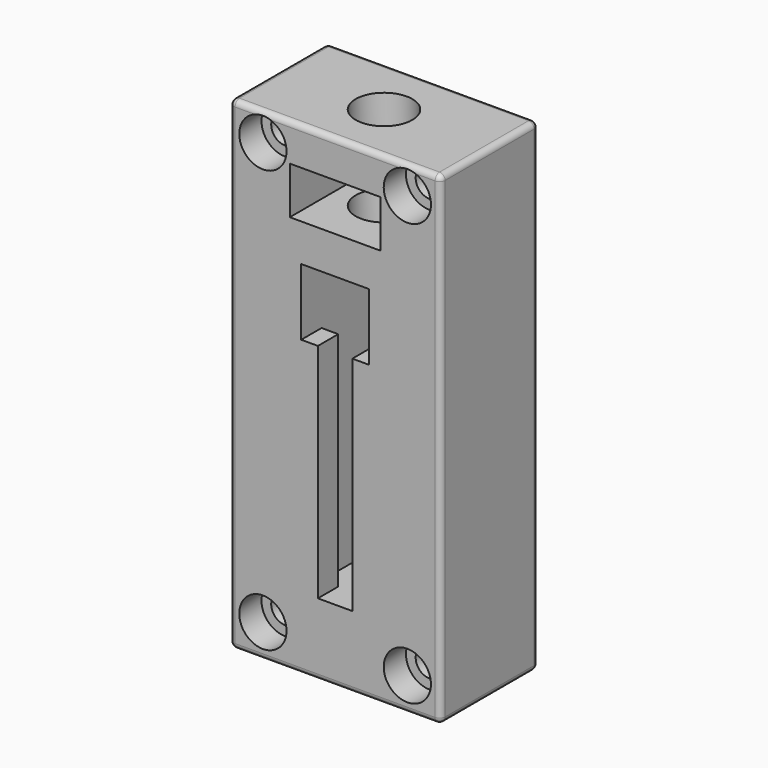
from build123d import *

# Parameters (mm, degrees)
F0_W         = 16.3
F0_H         = 8.5
F1_DEPTH     = 22
F2_R         = 5.1
F3_DEPTH     = 22
F4_W         = 3
F4_H         = 12.2
F4_W_2       = 9.2
F5_DEPTH     = 40
F6_R         = 2.5
F7_DEPTH     = 22.001
F6_R_2       = 4.25
F8_DEPTH     = 5
F9_T1_DEPTH  = 85
F9_T3_DEPTH  = 36
F9_T5_DEPTH  = 20
F9_S9_W      = 1
F9_S9_H      = 1
F9_T10_DEPTH = 1
F9_S15_W     = 1
F9_S15_H     = 1
F9_T16_DEPTH = 1
F9_S21_W     = 1
F9_S21_H     = 1
F9_T22_DEPTH = 1
F9_S27_W     = 1
F9_S27_H     = 1
F9_T28_DEPTH = 1
F9_S33_W     = 1
F9_S33_H     = 1
F9_T34_DEPTH = 1
F9_S39_W     = 1
F9_S39_H     = 1
F9_T40_DEPTH = 1
F9_S45_W     = 1
F9_S45_H     = 1
F9_T46_DEPTH = 1
F9_S51_W     = 1
F9_S51_H     = 1
F9_T52_DEPTH = 1


# Not quite as in the source:
# - a fillet or chamfer that OpenCascade refuses, or shapes differently, is made with other operations: its cross-section is extruded or revolved along the edge and cut away or added


with BuildPart() as f1:
    # F0 (on Front) → F1 (new body)
    with BuildSketch(Plane.XZ):
        Polygon((-19, 32), (-6.1, 32), (6.1, 32), (19, 32), (19, 54), (-19, 54), align=None)
        with Locations((0, 43)):
            Rectangle(F0_W, F0_H, mode=Mode.SUBTRACT)
        Polygon((-3.1, -20), (-3.1, 20), (-6.1, 20), (-6.1, 32), (-19, 32), (-19, -33), (19, -33), (19, 32), (6.1, 32), (6.1, 20), (3.1, 20), (3.1, -20), align=None)
    extrude(amount=F1_DEPTH)

    # F2 (on face) → F3 (cut, through all)
    with BuildSketch(Plane.XY.offset(54)):
        with Locations((0, -11)):
            Circle(F2_R)
    extrude(amount=-F3_DEPTH, mode=Mode.SUBTRACT)

    # F4 (on face) → F5 (cut)
    with BuildSketch(Plane.XY.offset(20)):
        with Locations((-4.6, -11.319772105)):
            Rectangle(F4_W, F4_H)
        with Locations((1.5, -11.319772105)):
            Rectangle(F4_W_2, F4_H)
    extrude(amount=-F5_DEPTH, mode=Mode.SUBTRACT)

    # F6 (on face) → F7 (cut, through all)
    with BuildSketch(Plane.XZ.offset(22)):
        with Locations((-13, 49)):
            Circle(F6_R)
        with Locations((13, 49)):
            Circle(F6_R)
        with Locations((-13, -27)):
            Circle(F6_R)
        with Locations((13, -27)):
            Circle(F6_R)
    extrude(amount=-F7_DEPTH, mode=Mode.SUBTRACT)

    # F6 (on face) → F8 (cut)
    with BuildSketch(Plane.XZ.offset(22)):
        with Locations((-13, 49)):
            Circle(F6_R_2)
        with Locations((-13, 49)):
            Circle(F6_R, mode=Mode.SUBTRACT)
        with Locations((13, 49)):
            Circle(F6_R_2)
        with Locations((13, 49)):
            Circle(F6_R, mode=Mode.SUBTRACT)
        with Locations((13, -27)):
            Circle(F6_R_2)
        with Locations((13, -27)):
            Circle(F6_R, mode=Mode.SUBTRACT)
        with Locations((-13, -27)):
            Circle(F6_R_2)
        with Locations((-13, -27)):
            Circle(F6_R, mode=Mode.SUBTRACT)
    extrude(amount=-F8_DEPTH, mode=Mode.SUBTRACT)

    # F9: fillet of radius 1 on 12 edges, made by hand

    # F9_s2 → F9_t1 (cut)
    with BuildSketch(Plane.XY.offset(-32)):
        with BuildLine():
            ThreePointArc((18, -22), (18.7071067812, -21.7071067812), (19, -21))
            Line((19, -21), (19, -22))
            Line((19, -22), (18, -22))
        make_face()
        with BuildLine():
            ThreePointArc((-18, -22), (-18.7071067812, -21.7071067812), (-19, -21))
            Line((-19, -21), (-19, -22))
            Line((-19, -22), (-18, -22))
        make_face()
        with BuildLine():
            ThreePointArc((-18, 0), (-18.7071067812, -0.2928932188), (-19, -1))
            Line((-19, -1), (-19, 0))
            Line((-19, 0), (-18, 0))
        make_face()
        with BuildLine():
            ThreePointArc((18, 0), (18.7071067812, -0.2928932188), (19, -1))
            Line((19, -1), (19, 0))
            Line((19, 0), (18, 0))
        make_face()
    extrude(amount=F9_T1_DEPTH, mode=Mode.SUBTRACT)

    # F9_s4 → F9_t3 (cut)
    with BuildSketch(Plane.YZ.offset(-18)):
        with BuildLine():
            ThreePointArc((-22, 53), (-21.7071067812, 53.7071067812), (-21, 54))
            Line((-21, 54), (-22, 54))
            Line((-22, 54), (-22, 53))
        make_face()
        with BuildLine():
            ThreePointArc((-22, -32), (-21.7071067812, -32.7071067812), (-21, -33))
            Line((-21, -33), (-22, -33))
            Line((-22, -33), (-22, -32))
        make_face()
        with BuildLine():
            ThreePointArc((0, 53), (-0.2928932188, 53.7071067812), (-1, 54))
            Line((-1, 54), (0, 54))
            Line((0, 54), (0, 53))
        make_face()
        with BuildLine():
            ThreePointArc((0, -32), (-0.2928932188, -32.7071067812), (-1, -33))
            Line((-1, -33), (0, -33))
            Line((0, -33), (0, -32))
        make_face()
    extrude(amount=F9_T3_DEPTH, mode=Mode.SUBTRACT)

    # F9_s6 → F9_t5 (cut)
    with BuildSketch(Plane.XZ.offset(1)):
        with BuildLine():
            ThreePointArc((19, -32), (18.7071067812, -32.7071067812), (18, -33))
            Line((18, -33), (19, -33))
            Line((19, -33), (19, -32))
        make_face()
        with BuildLine():
            ThreePointArc((18, 54), (18.7071067812, 53.7071067812), (19, 53))
            Line((19, 53), (19, 54))
            Line((19, 54), (18, 54))
        make_face()
        with BuildLine():
            ThreePointArc((-18, 54), (-18.7071067812, 53.7071067812), (-19, 53))
            Line((-19, 53), (-19, 54))
            Line((-19, 54), (-18, 54))
        make_face()
        with BuildLine():
            ThreePointArc((-19, -32), (-18.7071067812, -32.7071067812), (-18, -33))
            Line((-18, -33), (-19, -33))
            Line((-19, -33), (-19, -32))
        make_face()
    extrude(amount=F9_T5_DEPTH, mode=Mode.SUBTRACT)


with BuildPart() as f9_tool8:
    # F9_s9 → F9_t10 (new body)
    with BuildSketch(Plane.XZ.offset(21)):
        with Locations((18.5, -32.5)):
            Rectangle(F9_S9_W, F9_S9_H)
    extrude(amount=F9_T10_DEPTH)

    # F9_s11 → F9_t12 (revolve, cut)
    with BuildSketch(Plane(origin=(18, -21, -32), x_dir=(-0.7071067812, 0, 0.7071067812), z_dir=(0.7071067812, 0, 0.7071067812))):
        with BuildLine():
            ThreePointArc((0, -1), (1, 0), (0, 1))
            Line((0, 1), (0, -1))
        make_face()
    revolve(axis=Axis((18, -21, -32), (0, -1, 0)), mode=Mode.SUBTRACT)


with BuildPart() as f1_1:
    add(f1.part)

    # F9_t7: cut F9_tool8
    add(f9_tool8.part, mode=Mode.SUBTRACT)


with BuildPart() as f9_tool14:
    # F9_s15 → F9_t16 (new body)
    with BuildSketch(Plane.XY.offset(53)):
        with Locations((18.5, -21.5)):
            Rectangle(F9_S15_W, F9_S15_H)
    extrude(amount=F9_T16_DEPTH)

    # F9_s17 → F9_t18 (revolve, cut)
    with BuildSketch(Plane(origin=(18, -21, 53), x_dir=(-0.7071067812, 0.7071067812, 0), z_dir=(0.7071067812, 0.7071067812, 0))):
        with BuildLine():
            ThreePointArc((0, -1), (1, 0), (0, 1))
            Line((0, 1), (0, -1))
        make_face()
    revolve(axis=Axis((18, -21, 53), (0, 0, 1)), mode=Mode.SUBTRACT)


with BuildPart() as f1_2:
    add(f1_1.part)

    # F9_t13: cut F9_tool14
    add(f9_tool14.part, mode=Mode.SUBTRACT)


with BuildPart() as f9_tool20:
    # F9_s21 → F9_t22 (new body)
    with BuildSketch(Plane.XY.offset(53)):
        with Locations((-18.5, -21.5)):
            Rectangle(F9_S21_W, F9_S21_H)
    extrude(amount=F9_T22_DEPTH)

    # F9_s23 → F9_t24 (revolve, cut)
    with BuildSketch(Plane(origin=(-18, -21, 53), x_dir=(0.7071067812, 0.7071067812, 0), z_dir=(0.7071067812, -0.7071067812, 0))):
        with BuildLine():
            ThreePointArc((0, -1), (1, 0), (0, 1))
            Line((0, 1), (0, -1))
        make_face()
    revolve(axis=Axis((-18, -21, 53), (0, 0, 1)), mode=Mode.SUBTRACT)


with BuildPart() as f1_3:
    add(f1_2.part)

    # F9_t19: cut F9_tool20
    add(f9_tool20.part, mode=Mode.SUBTRACT)


with BuildPart() as f9_tool26:
    # F9_s27 → F9_t28 (new body)
    with BuildSketch(Plane.XZ.offset(21)):
        with Locations((-18.5, -32.5)):
            Rectangle(F9_S27_W, F9_S27_H)
    extrude(amount=F9_T28_DEPTH)

    # F9_s29 → F9_t30 (revolve, cut)
    with BuildSketch(Plane(origin=(-18, -21, -32), x_dir=(0.7071067812, 0, 0.7071067812), z_dir=(0.7071067812, 0, -0.7071067812))):
        with BuildLine():
            ThreePointArc((0, -1), (1, 0), (0, 1))
            Line((0, 1), (0, -1))
        make_face()
    revolve(axis=Axis((-18, -21, -32), (0, -1, 0)), mode=Mode.SUBTRACT)


with BuildPart() as f1_4:
    add(f1_3.part)

    # F9_t25: cut F9_tool26
    add(f9_tool26.part, mode=Mode.SUBTRACT)


with BuildPart() as f9_tool32:
    # F9_s33 → F9_t34 (new body)
    with BuildSketch(Plane.XZ.offset(1)):
        with Locations((18.5, -32.5)):
            Rectangle(F9_S33_W, F9_S33_H)
    extrude(amount=-F9_T34_DEPTH)

    # F9_s35 → F9_t36 (revolve, cut)
    with BuildSketch(Plane(origin=(18, -1, -32), x_dir=(-0.7071067812, 0, 0.7071067812), z_dir=(-0.7071067812, 0, -0.7071067812))):
        with BuildLine():
            ThreePointArc((0, -1), (1, 0), (0, 1))
            Line((0, 1), (0, -1))
        make_face()
    revolve(axis=Axis((18, -1, -32), (0, 1, 0)), mode=Mode.SUBTRACT)


with BuildPart() as f1_5:
    add(f1_4.part)

    # F9_t31: cut F9_tool32
    add(f9_tool32.part, mode=Mode.SUBTRACT)


with BuildPart() as f9_tool38:
    # F9_s39 → F9_t40 (new body)
    with BuildSketch(Plane.XZ.offset(1)):
        with Locations((18.5, 53.5)):
            Rectangle(F9_S39_W, F9_S39_H)
    extrude(amount=-F9_T40_DEPTH)

    # F9_s41 → F9_t42 (revolve, cut)
    with BuildSketch(Plane(origin=(18, -1, 53), x_dir=(-0.7071067812, 0, -0.7071067812), z_dir=(0.7071067812, 0, -0.7071067812))):
        with BuildLine():
            ThreePointArc((0, -1), (1, 0), (0, 1))
            Line((0, 1), (0, -1))
        make_face()
    revolve(axis=Axis((18, -1, 53), (0, 1, 0)), mode=Mode.SUBTRACT)


with BuildPart() as f1_6:
    add(f1_5.part)

    # F9_t37: cut F9_tool38
    add(f9_tool38.part, mode=Mode.SUBTRACT)


with BuildPart() as f9_tool44:
    # F9_s45 → F9_t46 (new body)
    with BuildSketch(Plane.XZ.offset(1)):
        with Locations((-18.5, 53.5)):
            Rectangle(F9_S45_W, F9_S45_H)
    extrude(amount=-F9_T46_DEPTH)

    # F9_s47 → F9_t48 (revolve, cut)
    with BuildSketch(Plane(origin=(-18, -1, 53), x_dir=(0.7071067812, 0, -0.7071067812), z_dir=(0.7071067812, 0, 0.7071067812))):
        with BuildLine():
            ThreePointArc((0, -1), (1, 0), (0, 1))
            Line((0, 1), (0, -1))
        make_face()
    revolve(axis=Axis((-18, -1, 53), (0, 1, 0)), mode=Mode.SUBTRACT)


with BuildPart() as f1_7:
    add(f1_6.part)

    # F9_t43: cut F9_tool44
    add(f9_tool44.part, mode=Mode.SUBTRACT)


with BuildPart() as f9_tool50:
    # F9_s51 → F9_t52 (new body)
    with BuildSketch(Plane.XZ.offset(1)):
        with Locations((-18.5, -32.5)):
            Rectangle(F9_S51_W, F9_S51_H)
    extrude(amount=-F9_T52_DEPTH)

    # F9_s53 → F9_t54 (revolve, cut)
    with BuildSketch(Plane(origin=(-18, -1, -32), x_dir=(0.7071067812, 0, 0.7071067812), z_dir=(-0.7071067812, 0, 0.7071067812))):
        with BuildLine():
            ThreePointArc((0, -1), (1, 0), (0, 1))
            Line((0, 1), (0, -1))
        make_face()
    revolve(axis=Axis((-18, -1, -32), (0, 1, 0)), mode=Mode.SUBTRACT)


with BuildPart() as f1_8:
    add(f1_7.part)

    # F9_t49: cut F9_tool50
    add(f9_tool50.part, mode=Mode.SUBTRACT)


solid = f1_8.part
